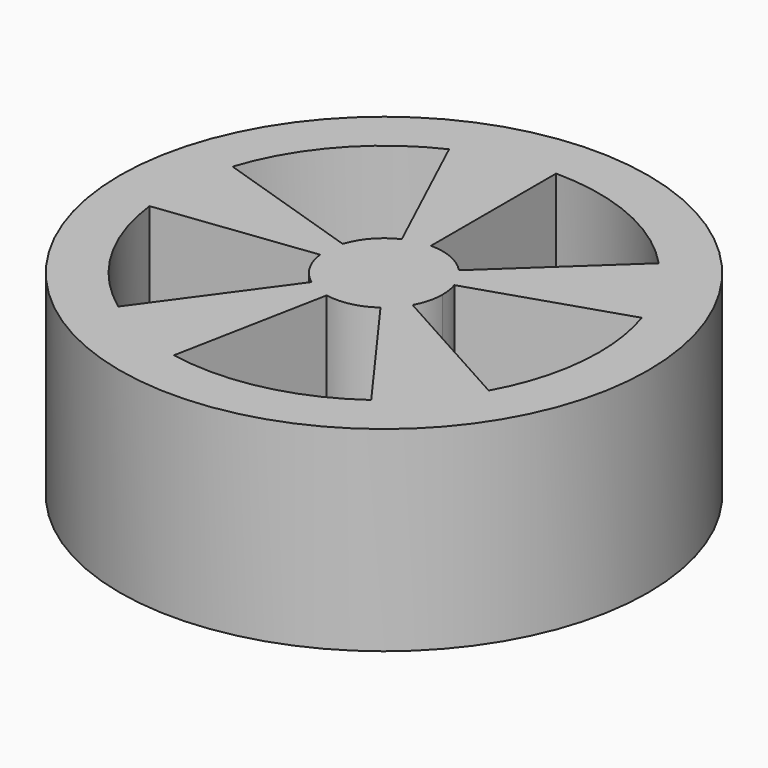
from build123d import *

# Parameters (mm, degrees)
F0_R     = 6.75
F1_DEPTH = 5
F3_DEPTH = 25


# Not quite as in the source:
# - a feature names something its author has since deleted; it is built from what else it names


with BuildPart() as f1:
    # F0 (on Top) → F1 (new body)
    with BuildSketch(Plane.XY):
        Circle(F0_R)
    extrude(amount=F1_DEPTH)

    # F2 (on face) → F3 (cut)
    with BuildSketch(Plane.XY.offset(5)):
        with BuildLine():
            Line((1.0970305524, 1.0229975401), (4.02115299, 3.7497858268))
            ThreePointArc((4.02115299, 3.7497858268), (2.192415253, 5.04220988), (0, 5.4982329084))
            Line((0, 5.4982329084), (0, 1.5))
            ThreePointArc((0, 1.5), (0.5981236034, 1.3755901116), (1.0970305524, 1.0229975401))
        make_face()
        with BuildLine():
            Line((-0.6339273926, 1.3594616806), (-2.3236536344, 4.9830912999))
            ThreePointArc((-2.3236536344, 4.9830912999), (-4.117932991, 3.6432393549), (-5.2291302357, 1.6990474077))
            Line((-5.2291302357, 1.6990474077), (-1.4265847744, 0.4635254916))
            ThreePointArc((-1.4265847744, 0.4635254916), (-1.1234335812, 0.9939300723), (-0.6339273926, 1.3594616806))
        make_face()
        with BuildLine():
            ThreePointArc((-5.4572499141, -0.6700660344), (-4.7374378048, -2.7905641295), (-3.2317802172, -4.448163862))
            Line((-3.2317802172, -4.448163862), (-0.8816778784, -1.2135254916))
            ThreePointArc((-0.8816778784, -1.2135254916), (-1.2924437407, -0.7613075444), (-1.4888192275, -0.1828040151))
            Line((-1.4888192275, -0.1828040151), (-5.4572499141, -0.6700660344))
        make_face()
        with BuildLine():
            ThreePointArc((-1.0491122976, -5.3972148839), (1.190035408, -5.3679028347), (3.2317802172, -4.448163862))
            Line((3.2317802172, -4.448163862), (0.8816778784, -1.2135254916))
            ThreePointArc((0.8816778784, -1.2135254916), (0.3246594209, -1.4644440107), (-0.2862134931, -1.4724407752))
            Line((-0.2862134931, -1.4724407752), (-1.0491122976, -5.3972148839))
        make_face()
        with BuildLine():
            ThreePointArc((4.8088628562, -2.6655962084), (5.3231012166, -1.3766475779), (5.4982329084, 0))
            ThreePointArc((5.4982329084, 0), (5.4305405375, 0.8601131237), (5.2291302357, 1.6990474077))
            Line((5.2291302357, 1.6990474077), (1.4265847744, 0.4635254916))
            ThreePointArc((1.4265847744, 0.4635254916), (1.4815325109, 0.2346516976), (1.5, 0))
            ThreePointArc((1.5, 0), (1.4522214606, -0.3755700061), (1.3119295607, -0.7272144304))
            Line((1.3119295607, -0.7272144304), (4.8088628562, -2.6655962084))
        make_face()
    extrude(amount=-F3_DEPTH, mode=Mode.SUBTRACT)


solid = f1.part
